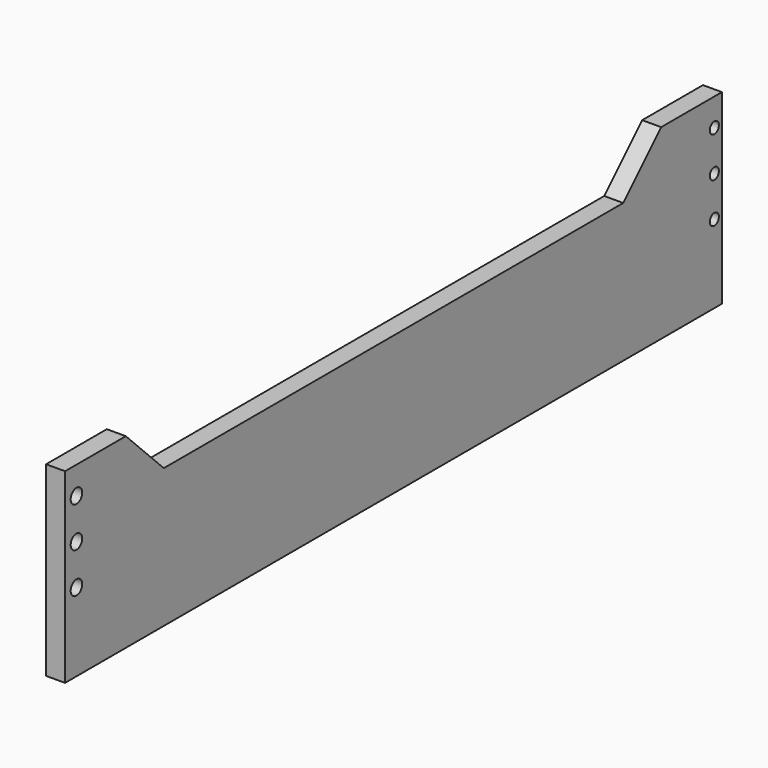
from build123d import *

# Parameters (mm, degrees)
F1_DEPTH = 6.35
F2_D     = 4.826
F3_D     = 3.81
F5_DEPTH = 25.4


# Not quite as in the source:
# - a feature names something its author has since deleted; it is built from what else it names


with BuildPart() as f1:
    # F0 (on Right) → F1 (new body)
    with BuildSketch(Plane.YZ):
        Polygon((274.6375, -12.7), (274.6375, 0), (274.6375, 53.8988), (0, 53.8988), (0, 0), (0, -12.7), align=None)
    extrude(amount=F1_DEPTH)

    # F2 (through all)
    with Locations(Plane(origin=(0, 0, 0), x_dir=(0, 1, 0), z_dir=(-1, 0, 0))):
        with Locations((4.7625, -40.4241), (4.7625, -26.9494), (4.7625, -13.4747)):
            Hole(F2_D / 2)

    # F3 (through all)
    with Locations(Plane(origin=(0, 0, 0), x_dir=(0, 1, 0), z_dir=(-1, 0, 0))):
        with Locations((271.4625, -40.4241), (271.4625, -26.9494), (271.4625, -13.4747)):
            Hole(F3_D / 2)

    # F4 (on face) → F5 (cut)
    with BuildSketch(Plane.YZ.offset(6.35)):
        Polygon((0, 53.8988), (0, 49.6316), (25.4, 49.6316), (41.275, 33.7566), (233.3625, 33.7566), (249.2375, 49.6316), (274.6375, 49.6316), (274.6375, 53.8988), align=None)
    extrude(amount=-F5_DEPTH, mode=Mode.SUBTRACT)


solid = f1.part
